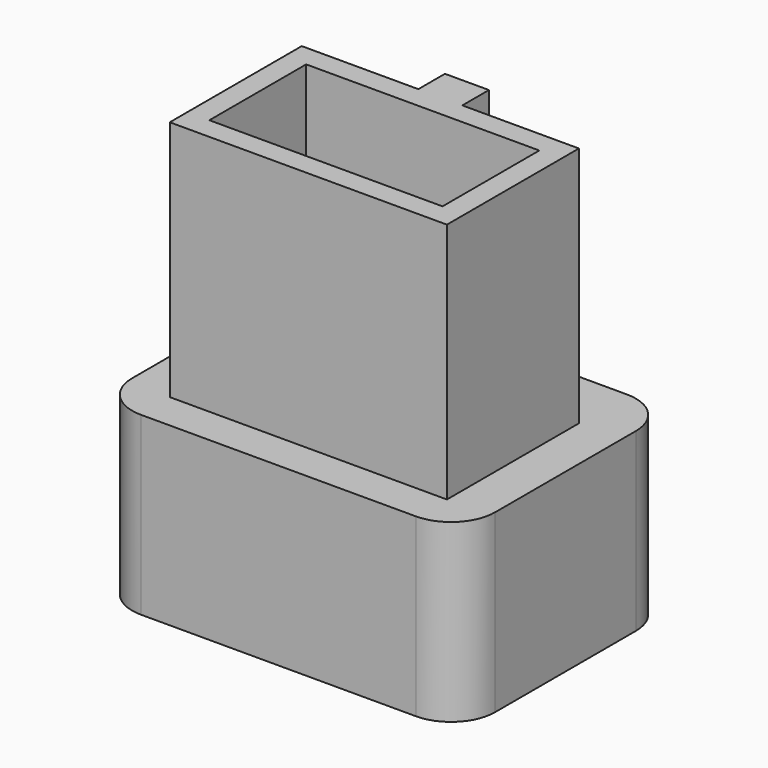
from build123d import *

# Parameters (mm, degrees)
F0_W        = 10.6
F0_H        = 5.5
F0_W_2      = 2
F0_H_2      = 1.512365222
F1_DEPTH    = 19
F0_W_3      = 16.5
F0_H_3      = 12
F2_DEPTH    = 8
F3_R        = 2
F4_T4_DEPTH = 2


# Not quite as in the source:
# - a fillet or chamfer that OpenCascade refuses, or shapes differently, is made with other operations: its cross-section is extruded or revolved along the edge and cut away or added


with BuildPart() as f1:
    # F0 (on Top) → F1 (new body)
    with BuildSketch(Plane.XY):
        Polygon((-6.3, -3.75), (6.3, -3.75), (6.3, 3.75), (1, 3.75), (-1, 3.75), (-6.3, 3.75), align=None)
        Rectangle(F0_W, F0_H, mode=Mode.SUBTRACT)
        with Locations((0, 4.506182611)):
            Rectangle(F0_W_2, F0_H_2)
    extrude(amount=F1_DEPTH)

    # F0 (on Top) → F2 (join)
    with BuildSketch(Plane.XY):
        with Locations((0, 0.5489425384)):
            Rectangle(F0_W_3, F0_H_3)
        Polygon((6.3, 3.75), (6.3, -3.75), (-6.3, -3.75), (-6.3, 3.75), (-1, 3.75), (-1, 5.262365222), (1, 5.262365222), (1, 3.75), align=None, mode=Mode.SUBTRACT)
    extrude(amount=F2_DEPTH)

    # F3
    f3_edges = [f1.edges().sort_by_distance(p)[0] for p in [
        (-8.25, -5.451057, 4),
        (8.25, -5.451057, 4),
        (8.25, 6.548943, 4),
        (-8.25, 6.548943, 4),
    ]]
    fillet(f3_edges, radius=F3_R)

    # F4: chamfer of 3 x 1.4 on 1 edges, made by hand


with BuildPart() as f4_tool2:
    # F4_s3 → F4_t4 (new body)
    with BuildSketch(Plane.YZ.offset(-1)):
        Polygon((6.662365222, 8), (5.262365222, 11), (5.262365222, 8), align=None)
    extrude(amount=F4_T4_DEPTH)

    split(bisect_by=Plane.XZ.offset(-6.5489425384), keep=Keep.TOP)


with BuildPart() as f1_1:
    add(f1.part)

    # F4_t1: union F4_tool2
    add(f4_tool2.part)


solid = f1_1.part
